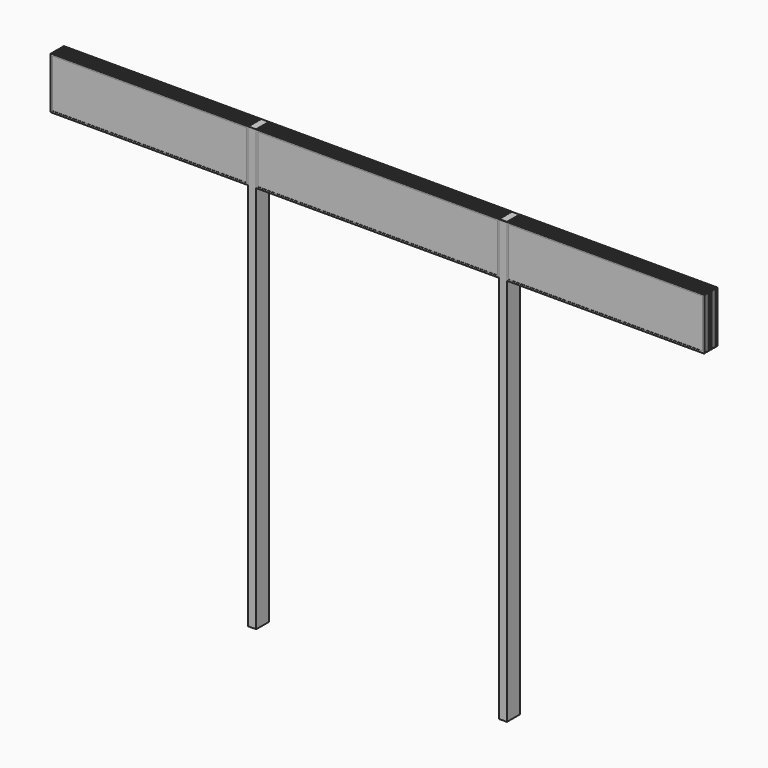
from build123d import *

# Parameters (mm, degrees)
F0_W      = 50
F0_H      = 2720
F1_DEPTH  = 100
F2_W      = 1220
F2_H      = 100
F3_DEPTH  = 320
F2_W_2    = 1500
F4_W      = 1200
F4_H      = 300
F4_W_2    = 1480
F5_DEPTH  = 100.001
F6_W      = 8
F6_H      = 2
F7_DEPTH  = 4040.001
F8_W      = 2
F8_H      = 8
F9_DEPTH  = 2720.001
F11_W     = 1480
F11_H     = 300
F12_DEPTH = 98
F11_W_2   = 1200
F13_R     = 1.9999
F13_2_R   = 1.9999
F13_3_R   = 1.9999
F13_4_R   = 1.9999
F13_5_R   = 1.9999


# Not quite as in the source:
# - a fillet or chamfer is up to 0.001 mm smaller than in the source, because OpenCascade refuses the exact size


with BuildPart() as f1:
    # F0 (on Front) → F1 (new body)
    with BuildSketch(Plane.XZ):
        with Locations((-775, -1360)):
            Rectangle(F0_W, F0_H)
    extrude(amount=F1_DEPTH)

    # F13 (radius 2 in the source; OpenCascade refuses exactly that, so slightly less here)
    f13_edges = [f1.edges().sort_by_distance(p)[0] for p in [
        (-750, -50, 0),
        (-800, -50, 0),
    ]]
    fillet(f13_edges, radius=F13_R)


with BuildPart() as f1b:
    # F0 (on Front) → F1, piece 2 (new body)
    with BuildSketch(Plane.XZ):
        with Locations((775, -1360)):
            Rectangle(F0_W, F0_H)
    extrude(amount=F1_DEPTH)

    # F13#2 (radius 2 in the source; OpenCascade refuses exactly that, so slightly less here)
    f13_2_edges = [f1b.edges().sort_by_distance(p)[0] for p in [
        (800, -50, 0),
        (750, -50, 0),
        (775, 0, 0),
        (775, -100, 0),
    ]]
    fillet(f13_2_edges, radius=F13_2_R)


with BuildPart() as f3:
    # F2 (on face) → F3 (new body)
    with BuildSketch(Plane.XY):
        with Locations((-1410, -50)):
            Rectangle(F2_W, F2_H)
    extrude(amount=-F3_DEPTH)


with BuildPart() as f3b:
    # F2 (on face) → F3, piece 2 (new body)
    with BuildSketch(Plane.XY):
        with Locations((0, -50)):
            Rectangle(F2_W_2, F2_H)
    extrude(amount=-F3_DEPTH)


with BuildPart() as f3c:
    # F2 (on face) → F3, piece 3 (new body)
    with BuildSketch(Plane.XY):
        with Locations((1410, -50)):
            Rectangle(F2_W, F2_H)
    extrude(amount=-F3_DEPTH)


with BuildPart() as f5_tool:
    # F4 (on face) → F5 (new body, through all)
    with BuildSketch(Plane.XZ.offset(100)):
        with Locations((-1410, -160)):
            Rectangle(F4_W, F4_H)
        with Locations((0, -160)):
            Rectangle(F4_W_2, F4_H)
        with Locations((1410, -160)):
            Rectangle(F4_W, F4_H)
    extrude(amount=-F5_DEPTH)


with BuildPart() as f3_1:
    add(f3.part)

    # F5: cut by f5_tool
    add(f5_tool.part, mode=Mode.SUBTRACT)


with BuildPart() as f3b_1:
    add(f3b.part)

    # F5: cut by f5_tool
    add(f5_tool.part, mode=Mode.SUBTRACT)


with BuildPart() as f3c_1:
    add(f3c.part)

    # F5: cut by f5_tool
    add(f5_tool.part, mode=Mode.SUBTRACT)


with BuildPart() as f7_tool:
    # F6 (on face) → F7 (new body, through all)
    with BuildSketch(Plane(origin=(-2020, 0, 0), x_dir=(0, -1, 0), z_dir=(-1, 0, 0))):
        with Locations((14, -1)):
            Rectangle(F6_W, F6_H)
        with Locations((32, -1)):
            Rectangle(F6_W, F6_H)
        with Locations((50, -1)):
            Rectangle(F6_W, F6_H)
        with Locations((68, -1)):
            Rectangle(F6_W, F6_H)
        with Locations((86, -1)):
            Rectangle(F6_W, F6_H)
        with Locations((86, -319)):
            Rectangle(F6_W, F6_H)
        with Locations((68, -319)):
            Rectangle(F6_W, F6_H)
        with Locations((14, -319)):
            Rectangle(F6_W, F6_H)
        with Locations((32, -319)):
            Rectangle(F6_W, F6_H)
        with Locations((50, -319)):
            Rectangle(F6_W, F6_H)
    extrude(amount=-F7_DEPTH)


with BuildPart() as f3_2:
    add(f3_1.part)

    # F7: cut by f7_tool
    add(f7_tool.part, mode=Mode.SUBTRACT)


with BuildPart() as f3b_2:
    add(f3b_1.part)

    # F7: cut by f7_tool
    add(f7_tool.part, mode=Mode.SUBTRACT)

    # F13#4 (radius 2 in the source; OpenCascade refuses exactly that, so slightly less here)
    f13_4_edges = [f3b_2.edges().sort_by_distance(p)[0] for p in [
        (750, -41, 0),
        (750, -23, 0),
        (750, -5, 0),
        (750, -59, 0),
        (750, -77, 0),
        (750, -95, 0),
        (750, -86, -2),
        (750, -68, -2),
        (750, -50, -2),
        (750, -32, -2),
        (750, -14, -2),
        (750, -95, -320),
        (750, -86, -318),
        (750, -77, -320),
        (750, -68, -318),
        (750, -59, -320),
        (750, -50, -318),
        (750, -41, -320),
        (750, -32, -318),
        (750, -23, -320),
        (750, -14, -318),
        (750, -5, -320),
        (-750, -5, -320),
        (-750, -23, -320),
        (-750, -32, -318),
        (-750, -41, -320),
        (-750, -50, -318),
        (-750, -59, -320),
        (-750, -68, -318),
        (-750, -77, -320),
        (-750, -86, -318),
        (-750, -95, -320),
        (-750, -14, -318),
        (-750, -95, 0),
        (-750, -77, 0),
        (-750, -59, 0),
        (-750, -68, -2),
        (-750, -86, -2),
        (-750, -50, -2),
        (-750, -41, 0),
        (-750, -32, -2),
        (-750, -23, 0),
        (-750, -14, -2),
        (-750, -5, 0),
    ]]
    fillet(f13_4_edges, radius=F13_4_R)


with BuildPart() as f3c_2:
    add(f3c_1.part)

    # F7: cut by f7_tool
    add(f7_tool.part, mode=Mode.SUBTRACT)


with BuildPart() as f9_tool:
    # F8 (on face) → F9 (new body, through all)
    with BuildSketch(Plane.XY):
        with Locations((-2019, -86)):
            Rectangle(F8_W, F8_H)
        with Locations((-2019, -68)):
            Rectangle(F8_W, F8_H)
        with Locations((-2019, -50)):
            Rectangle(F8_W, F8_H)
        with Locations((-2019, -32)):
            Rectangle(F8_W, F8_H)
        with Locations((-2019, -14)):
            Rectangle(F8_W, F8_H)
        with Locations((2019, -68)):
            Rectangle(F8_W, F8_H)
        with Locations((2019, -32)):
            Rectangle(F8_W, F8_H)
        with Locations((2019, -86)):
            Rectangle(F8_W, F8_H)
        with Locations((2019, -50)):
            Rectangle(F8_W, F8_H)
        with Locations((2019, -14)):
            Rectangle(F8_W, F8_H)
    extrude(amount=-F9_DEPTH)


with BuildPart() as f3_3:
    add(f3_2.part)

    # F9: cut by f9_tool
    add(f9_tool.part, mode=Mode.SUBTRACT)

    # F13#3 (radius 2 in the source; OpenCascade refuses exactly that, so slightly less here)
    f13_3_edges = [f3_3.edges().sort_by_distance(p)[0] for p in [
        (-800, -5, -320),
        (-800, -14, -318),
        (-800, -23, -320),
        (-800, -32, -318),
        (-800, -41, -320),
        (-800, -50, -318),
        (-800, -59, -320),
        (-800, -68, -318),
        (-800, -77, -320),
        (-800, -86, -318),
        (-800, -95, -320),
        (-2020, -95, -320),
        (-2018, -86, -318),
        (-2020, -77, -320),
        (-2018, -68, -318),
        (-2020, -59, -320),
        (-2018, -50, -318),
        (-2020, -41, -320),
        (-2018, -32, -318),
        (-2020, -23, -320),
        (-2018, -14, -318),
        (-2020, -5, -320),
        (-2020, -95, 0),
        (-2018, -86, -2),
        (-2020, -77, 0),
        (-2018, -68, -2),
        (-2020, -59, 0),
        (-2018, -50, -2),
        (-2020, -41, 0),
        (-2018, -32, -2),
        (-2020, -23, 0),
        (-2018, -14, -2),
        (-2020, -5, 0),
        (-800, -95, 0),
        (-800, -77, 0),
        (-800, -59, 0),
        (-800, -41, 0),
        (-800, -23, 0),
        (-800, -5, 0),
        (-800, -14, -2),
        (-800, -32, -2),
        (-800, -50, -2),
        (-800, -68, -2),
        (-800, -86, -2),
    ]]
    fillet(f13_3_edges, radius=F13_3_R)


with BuildPart() as f3c_3:
    add(f3c_2.part)

    # F9: cut by f9_tool
    add(f9_tool.part, mode=Mode.SUBTRACT)

    # F13#5 (radius 2 in the source; OpenCascade refuses exactly that, so slightly less here)
    f13_5_edges = [f3c_3.edges().sort_by_distance(p)[0] for p in [
        (2020, -5, 0),
        (2020, -23, 0),
        (2020, -41, 0),
        (2020, -59, 0),
        (2020, -77, 0),
        (2020, -95, 0),
        (2018, -86, -2),
        (2018, -68, -2),
        (2018, -50, -2),
        (2018, -32, -2),
        (2018, -14, -2),
        (800, -5, 0),
        (800, -23, 0),
        (800, -41, 0),
        (800, -59, 0),
        (800, -95, 0),
        (800, -77, 0),
        (800, -86, -2),
        (800, -68, -2),
        (800, -50, -2),
        (800, -32, -2),
        (800, -14, -2),
        (2020, -5, -320),
        (2018, -14, -318),
        (2020, -23, -320),
        (2018, -32, -318),
        (2020, -41, -320),
        (2018, -50, -318),
        (2020, -59, -320),
        (2018, -68, -318),
        (2020, -77, -320),
        (2018, -86, -318),
        (2020, -95, -320),
        (800, -5, -320),
        (800, -14, -318),
        (800, -23, -320),
        (800, -32, -318),
        (800, -41, -320),
        (800, -50, -318),
        (800, -59, -320),
        (800, -68, -318),
        (800, -77, -320),
        (800, -86, -318),
        (800, -95, -320),
    ]]
    fillet(f13_5_edges, radius=F13_5_R)


with BuildPart() as f12:
    # F11 (on offset) → F12 (new body, through all)
    with BuildSketch(Plane(origin=(0, -1, 0), x_dir=(-1, 0, 0), z_dir=(0, 1, 0))):
        with Locations((0, -160)):
            Rectangle(F11_W, F11_H)
    extrude(amount=-F12_DEPTH)


with BuildPart() as f12b:
    # F11 (on offset) → F12, piece 2 (new body, through all)
    with BuildSketch(Plane(origin=(0, -1, 0), x_dir=(-1, 0, 0), z_dir=(0, 1, 0))):
        with Locations((-1410, -160)):
            Rectangle(F11_W_2, F11_H)
    extrude(amount=-F12_DEPTH)


with BuildPart() as f12c:
    # F11 (on offset) → F12, piece 3 (new body, through all)
    with BuildSketch(Plane(origin=(0, -1, 0), x_dir=(-1, 0, 0), z_dir=(0, 1, 0))):
        with Locations((1410, -160)):
            Rectangle(F11_W_2, F11_H)
    extrude(amount=-F12_DEPTH)


solid = Compound([f1.part, f1b.part, f3b_2.part, f3_3.part, f3c_3.part, f12.part, f12b.part, f12c.part])
